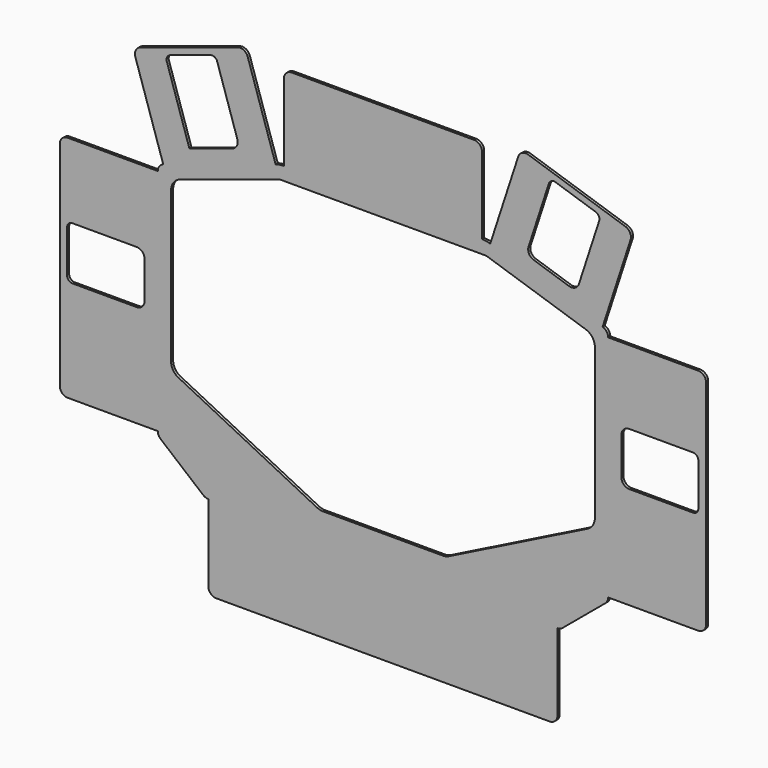
from build123d import *

# Parameters (mm, degrees)
F1_DEPTH = 1


# Not quite as in the source:
# - a feature names something its author has since deleted; it is built from what else it names


with BuildPart() as f1:
    # F0 (on Front) → F1 (new body)
    with BuildSketch(Plane.XZ):
        with BuildLine():
            ThreePointArc((83.920553199, 4.6283250442), (84.7167682637, 5.6605226942), (85, 6.932988883))
            Line((85, 6.932988883), (85, 25.527864045))
            Line((85, 25.527864045), (85, 45.527864045))
            Line((85, 45.527864045), (85, 55.527864045))
            Line((85, 55.527864045), (85, 65.527864045))
            Line((85, 65.527864045), (85, 90.527864045))
            Line((85, 90.527864045), (85, 93.3506543745))
            ThreePointArc((85, 93.3506543745), (84.4279811983, 95.1127290894), (82.9300617995, 96.202843893))
            Line((82.9300617995, 96.202843893), (71.5072983948, 99.9276580467))
            Line((71.5072983948, 99.9276580467), (62, 103.027864045))
            Line((62, 103.027864045), (52.4927016052, 106.1280700433))
            Line((52.4927016052, 106.1280700433), (40.5109515892, 110.0351624398))
            ThreePointArc((40.5109515892, 110.0351624398), (38.9803022245, 110.4039205441), (37.4107455909, 110.527864045))
            Line((37.4107455909, 110.527864045), (37.4107455909, 139.527864045))
            ThreePointArc((37.4107455909, 139.527864045), (36.5320659345, 141.6491843886), (34.4107455909, 142.527864045))
            Line((34.4107455909, 142.527864045), (0, 142.527864045))
            Line((0, 142.527864045), (-34.4107455909, 142.527864045))
            ThreePointArc((-34.4107455909, 142.527864045), (-36.5320659345, 141.6491843886), (-37.4107455909, 139.527864045))
            Line((-37.4107455909, 139.527864045), (-37.4107455909, 110.527864045))
            ThreePointArc((-37.4107455909, 110.527864045), (-38.9803022245, 110.4039205441), (-40.5109515892, 110.0351624398))
            Line((-40.5109515892, 110.0351624398), (-52.4927016052, 106.1280700433))
            Line((-52.4927016052, 106.1280700433), (-62, 103.027864045))
            Line((-62, 103.027864045), (-71.5072983948, 99.9276580467))
            Line((-71.5072983948, 99.9276580467), (-82.9300617995, 96.202843893))
            ThreePointArc((-82.9300617995, 96.202843893), (-84.4279811983, 95.1127290894), (-85, 93.3506543745))
            Line((-85, 93.3506543745), (-85, 90.527864045))
            Line((-85, 90.527864045), (-85, 65.527864045))
            Line((-85, 65.527864045), (-85, 45.527864045))
            Line((-85, 45.527864045), (-85, 25.527864045))
            Line((-85, 25.527864045), (-85, 6.932988883))
            ThreePointArc((-85, 6.932988883), (-84.7167682637, 5.6605226942), (-83.920553199, 4.6283250442))
            Line((-83.920553199, 4.6283250442), (-67.8344033934, -8.7767997938))
            ThreePointArc((-67.8344033934, -8.7767997938), (-66.9351259857, -9.292950688), (-65.9138501945, -9.472135955))
            Line((-65.9138501945, -9.472135955), (-65.9138501945, -38.472135955))
            ThreePointArc((-65.9138501945, -38.472135955), (-65.035170538, -40.5934562986), (-62.9138501945, -41.472135955))
            Line((-62.9138501945, -41.472135955), (0, -41.472135955))
            Line((0, -41.472135955), (62.9138501945, -41.472135955))
            ThreePointArc((62.9138501945, -41.472135955), (65.035170538, -40.5934562986), (65.9138501945, -38.472135955))
            Line((65.9138501945, -38.472135955), (65.9138501945, -9.472135955))
            ThreePointArc((65.9138501945, -9.472135955), (66.9351259857, -9.292950688), (67.8344033934, -8.7767997938))
            Line((67.8344033934, -8.7767997938), (83.920553199, 4.6283250442))
        make_face()
        with BuildLine():
            ThreePointArc((38.9901511122, 105.4658922946), (39.3764477711, 105.3887881754), (39.7554757946, 105.2815132424))
            Line((39.7554757946, 105.2815132424), (76.5501029992, 93.2832652409))
            ThreePointArc((76.5501029992, 93.2832652409), (77.9421273317, 92.5723733654), (79.0466353305, 91.466407235))
            ThreePointArc((79.0466353305, 91.466407235), (79.7556900999, 90.0734462394), (80, 88.5296160435))
            Line((80, 88.5296160435), (80, 31.7082039325))
            ThreePointArc((80, 31.7082039325), (79.8096917889, 30.3418712879), (79.2532540418, 29.0795483719))
            ThreePointArc((79.2532540418, 29.0795483719), (78.3730446274, 28.0173273508), (77.2360679775, 27.2360679775))
            Line((77.2360679775, 27.2360679775), (24.8753882025, 1.05572809))
            ThreePointArc((24.8753882025, 1.05572809), (24.3431697998, 0.8271304186), (23.7880848277, 0.6616190977))
            ThreePointArc((23.7880848277, 0.6616190977), (23.2175828225, 0.5614153774), (22.639320225, 0.527864045))
            Line((22.639320225, 0.527864045), (0, 0.527864045))
            Line((0, 0.527864045), (-22.639320225, 0.527864045))
            ThreePointArc((-22.639320225, 0.527864045), (-23.2175828225, 0.5614153774), (-23.7880848277, 0.6616190977))
            ThreePointArc((-23.7880848277, 0.6616190977), (-24.3431697998, 0.8271304186), (-24.8753882025, 1.05572809))
            Line((-24.8753882025, 1.05572809), (-77.2360679775, 27.2360679775))
            ThreePointArc((-77.2360679775, 27.2360679775), (-78.3730446274, 28.0173273508), (-79.2532540418, 29.0795483719))
            ThreePointArc((-79.2532540418, 29.0795483719), (-79.8096917889, 30.3418712879), (-80, 31.7082039325))
            Line((-80, 31.7082039325), (-80, 88.5296160435))
            ThreePointArc((-80, 88.5296160435), (-79.7556900999, 90.0734462394), (-79.0466353305, 91.466407235))
            ThreePointArc((-79.0466353305, 91.466407235), (-77.9421273317, 92.5723733654), (-76.5501029992, 93.2832652409))
            Line((-76.5501029992, 93.2832652409), (-39.7554757946, 105.2815132424))
            ThreePointArc((-39.7554757946, 105.2815132424), (-39.3764477711, 105.3887881754), (-38.9901511122, 105.4658922946))
            ThreePointArc((-38.9901511122, 105.4658922946), (-38.5989834865, 105.5123470296), (-38.2053727955, 105.527864045))
            Line((-38.2053727955, 105.527864045), (0, 105.527864045))
            Line((0, 105.527864045), (38.2053727955, 105.527864045))
            ThreePointArc((38.2053727955, 105.527864045), (38.5989834865, 105.5123470296), (38.9901511122, 105.4658922946))
        make_face(mode=Mode.SUBTRACT)
        with BuildLine():
            Line((71.5072983948, 99.9276580467), (82.9300617995, 96.202843893))
            Line((82.9300617995, 96.202843893), (93.4707621937, 128.5276584354))
            ThreePointArc((93.4707621937, 128.5276584354), (93.2930282304, 130.8168697792), (91.5486344748, 132.3099097533))
            Line((91.5486344748, 132.3099097533), (54.8339033014, 144.2821047011))
            ThreePointArc((54.8339033014, 144.2821047011), (52.5446919576, 144.1043707378), (51.0516519835, 142.3599769822))
            Line((51.0516519835, 142.3599769822), (40.5109515892, 110.0351624398))
            Line((40.5109515892, 110.0351624398), (52.4927016052, 106.1280700433))
            Line((52.4927016052, 106.1280700433), (62, 103.027864045))
            Line((62, 103.027864045), (71.5072983948, 99.9276580467))
        make_face()
        with BuildLine():
            Line((70.2052118755, 105.6113690436), (63.5501029992, 107.7815132424))
            Line((63.5501029992, 107.7815132424), (56.8949941228, 109.9516574412))
            ThreePointArc((56.8949941228, 109.9516574412), (55.1506003672, 111.4446974153), (54.9728664038, 113.7339087592))
            Line((54.9728664038, 113.7339087592), (61.7933196001, 134.6499652278))
            Line((61.7933196001, 134.6499652278), (62.6224189104, 137.192536446))
            ThreePointArc((62.6224189104, 137.192536446), (63.6177788931, 138.3554656164), (65.143919789, 138.4739549253))
            Line((65.143919789, 138.4739549253), (80.3555972207, 133.513625328))
            ThreePointArc((80.3555972207, 133.513625328), (81.5185263911, 132.5182653453), (81.6370157, 130.9921244494))
            Line((81.6370157, 130.9921244494), (80.8079163897, 128.4495532311))
            Line((80.8079163897, 128.4495532311), (73.9874631935, 107.5334967625))
            ThreePointArc((73.9874631935, 107.5334967625), (72.4944232194, 105.789103007), (70.2052118755, 105.6113690436))
        make_face(mode=Mode.SUBTRACT)
        with BuildLine():
            Line((85, 25.527864045), (85, 6.932988883))
            Line((85, 6.932988883), (114, 6.932988883))
            Line((114, 6.932988883), (117, 6.932988883))
            Line((117, 6.932988883), (119, 6.932988883))
            ThreePointArc((119, 6.932988883), (121.1213203436, 7.8116685394), (122, 9.932988883))
            Line((122, 9.932988883), (122, 90.3506543745))
            ThreePointArc((122, 90.3506543745), (121.1213203436, 92.4719747181), (119, 93.3506543745))
            Line((119, 93.3506543745), (117, 93.3506543745))
            Line((117, 93.3506543745), (114, 93.3506543745))
            Line((114, 93.3506543745), (85, 93.3506543745))
            Line((85, 93.3506543745), (85, 90.527864045))
            Line((85, 90.527864045), (85, 65.527864045))
            Line((85, 65.527864045), (85, 55.527864045))
            Line((85, 55.527864045), (85, 45.527864045))
            Line((85, 45.527864045), (85, 25.527864045))
        make_face()
        with BuildLine():
            Line((90.0046601892, 48.527864045), (90.0046601892, 55.527864045))
            Line((90.0046601892, 55.527864045), (90.0046601892, 62.527864045))
            ThreePointArc((90.0046601892, 62.527864045), (90.8833398456, 64.6491843886), (93.0046601892, 65.527864045))
            Line((93.0046601892, 65.527864045), (117.0514340997, 65.527864045))
            ThreePointArc((117.0514340997, 65.527864045), (118.465647662, 64.9420776074), (119.0514340997, 63.527864045))
            Line((119.0514340997, 63.527864045), (119.0514340997, 55.527864045))
            Line((119.0514340997, 55.527864045), (119.0514340997, 47.527864045))
            ThreePointArc((119.0514340997, 47.527864045), (118.465647662, 46.1136504826), (117.0514340997, 45.527864045))
            Line((117.0514340997, 45.527864045), (93.0046601892, 45.527864045))
            ThreePointArc((93.0046601892, 45.527864045), (90.8833398456, 46.4065437014), (90.0046601892, 48.527864045))
        make_face(mode=Mode.SUBTRACT)
        with BuildLine():
            Line((-114, 6.932988883), (-85, 6.932988883))
            Line((-85, 6.932988883), (-85, 25.527864045))
            Line((-85, 25.527864045), (-85, 45.527864045))
            Line((-85, 45.527864045), (-85, 65.527864045))
            Line((-85, 65.527864045), (-85, 90.527864045))
            Line((-85, 90.527864045), (-85, 93.3506543745))
            Line((-85, 93.3506543745), (-114, 93.3506543745))
            Line((-114, 93.3506543745), (-117, 93.3506543745))
            Line((-117, 93.3506543745), (-119, 93.3506543745))
            ThreePointArc((-119, 93.3506543745), (-121.1213203436, 92.4719747181), (-122, 90.3506543745))
            Line((-122, 90.3506543745), (-122, 9.932988883))
            ThreePointArc((-122, 9.932988883), (-121.1213203436, 7.8116685394), (-119, 6.932988883))
            Line((-119, 6.932988883), (-117, 6.932988883))
            Line((-117, 6.932988883), (-114, 6.932988883))
        make_face()
        with BuildLine():
            Line((-90, 55.527864045), (-90, 48.527864045))
            ThreePointArc((-90, 48.527864045), (-90.8786796564, 46.4065437014), (-93, 45.527864045))
            Line((-93, 45.527864045), (-108.2668378949, 45.527864045))
            Line((-108.2668378949, 45.527864045), (-115, 45.527864045))
            Line((-115, 45.527864045), (-116, 45.527864045))
            Line((-116, 45.527864045), (-117.232930243, 45.527864045))
            ThreePointArc((-117.232930243, 45.527864045), (-118.6471438054, 46.1136504826), (-119.232930243, 47.527864045))
            Line((-119.232930243, 47.527864045), (-119.232930243, 55.527864045))
            Line((-119.232930243, 55.527864045), (-119.232930243, 63.527864045))
            ThreePointArc((-119.232930243, 63.527864045), (-118.6471438054, 64.9420776074), (-117.232930243, 65.527864045))
            Line((-117.232930243, 65.527864045), (-116, 65.527864045))
            Line((-116, 65.527864045), (-115, 65.527864045))
            Line((-115, 65.527864045), (-113.2454946637, 65.527864045))
            Line((-113.2454946637, 65.527864045), (-93, 65.527864045))
            ThreePointArc((-93, 65.527864045), (-90.8786796564, 64.6491843886), (-90, 62.527864045))
            Line((-90, 62.527864045), (-90, 55.527864045))
        make_face(mode=Mode.SUBTRACT)
        with BuildLine():
            Line((-93.4707621937, 128.5276584354), (-82.9300617995, 96.202843893))
            Line((-82.9300617995, 96.202843893), (-71.5072983948, 99.9276580467))
            Line((-71.5072983948, 99.9276580467), (-62, 103.027864045))
            Line((-62, 103.027864045), (-52.4927016052, 106.1280700433))
            Line((-52.4927016052, 106.1280700433), (-40.5109515892, 110.0351624398))
            Line((-40.5109515892, 110.0351624398), (-51.0516519835, 142.3599769822))
            ThreePointArc((-51.0516519835, 142.3599769822), (-52.5446919576, 144.1043707378), (-54.8339033014, 144.2821047011))
            Line((-54.8339033014, 144.2821047011), (-91.5486344748, 132.3099097533))
            ThreePointArc((-91.5486344748, 132.3099097533), (-93.2930282304, 130.8168697792), (-93.4707621937, 128.5276584354))
        make_face()
        with BuildLine():
            Line((-56.8949941228, 109.9516574412), (-63.5501029992, 107.7815132424))
            Line((-63.5501029992, 107.7815132424), (-70.2052118755, 105.6113690436))
            Line((-70.2052118755, 105.6113690436), (-73.057401394, 104.6813072441))
            Line((-73.057401394, 104.6813072441), (-73.9874631935, 107.5334967625))
            Line((-73.9874631935, 107.5334967625), (-80.4169615485, 127.2506250513))
            Line((-80.4169615485, 127.2506250513), (-81.5932293444, 130.8578462922))
            ThreePointArc((-81.5932293444, 130.8578462922), (-81.4747400355, 132.3839871881), (-80.3118108651, 133.3793471708))
            Line((-80.3118108651, 133.3793471708), (-65.1001334334, 138.3396767681))
            ThreePointArc((-65.1001334334, 138.3396767681), (-63.5739925375, 138.2211874592), (-62.5786325548, 137.0582582888))
            Line((-62.5786325548, 137.0582582888), (-61.7933196001, 134.6499652278))
            Line((-61.7933196001, 134.6499652278), (-54.9728664038, 113.7339087592))
            ThreePointArc((-54.9728664038, 113.7339087592), (-55.1506003672, 111.4446974153), (-56.8949941228, 109.9516574412))
        make_face(mode=Mode.SUBTRACT)
    extrude(amount=F1_DEPTH)


solid = f1.part
